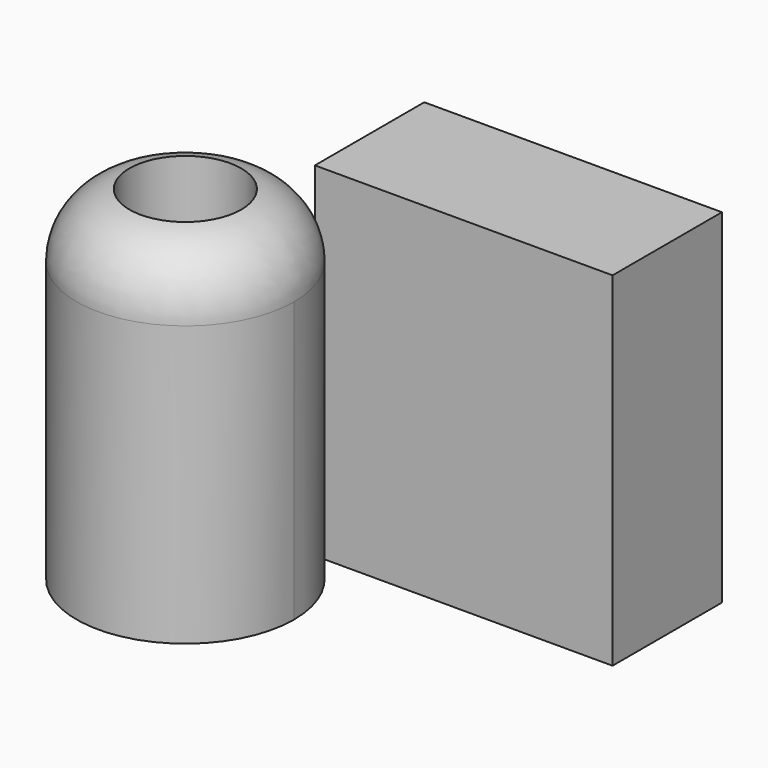
from build123d import *

# Parameters (mm, degrees)
F1_DEPTH = 39.5
F0_W     = 34.2074480574
F0_H     = 15.712268627
F2_R     = 6.4243054604
F3_DEPTH = 25


# Not quite as in the source:
# - a fillet or chamfer that OpenCascade refuses, or shapes differently, is made with other operations: its cross-section is extruded or revolved along the edge and cut away or added


with BuildPart() as f1:
    # F0 (on Top) → F1 (new body)
    with BuildSketch(Plane.XY):
        with BuildLine():
            ThreePointArc((6.2135610063, 10.8462739971), (-10.8147934002, -6.268193018), (12.5, 0))
            ThreePointArc((12.5, 0), (10.8147934002, 6.268193018), (6.2135610063, 10.8462739971))
        make_face()
    extrude(amount=F1_DEPTH)

    # F2 (on face) → F3 (cut)
    with BuildSketch(Plane.XY.offset(39.5)):
        Circle(F2_R)
    extrude(amount=-F3_DEPTH, mode=Mode.SUBTRACT)

    # F4: fillet of radius 7.4840620434 on 1 edges, made by hand

    # F4_s1 → F4_t2 (revolve, cut)
    with BuildSketch(Plane.XZ):
        with BuildLine():
            ThreePointArc((12.5, 32.1496472436), (10.7844513893, 36.9178164358), (6.4243054604, 39.5))
            Line((6.4243054604, 39.5), (12.5, 39.5))
            Line((12.5, 39.5), (12.5, 32.1496472436))
        make_face()
    revolve(axis=Axis((0, 0, 39.5), (0, 0, -1)), mode=Mode.SUBTRACT)


with BuildPart() as f1b:
    # F0 (on Top) → F1, piece 2 (new body)
    with BuildSketch(Plane.XY):
        with Locations((23.317285035, 18.7024083106)):
            Rectangle(F0_W, F0_H)
    extrude(amount=F1_DEPTH)


solid = Compound([f1.part, f1b.part])
